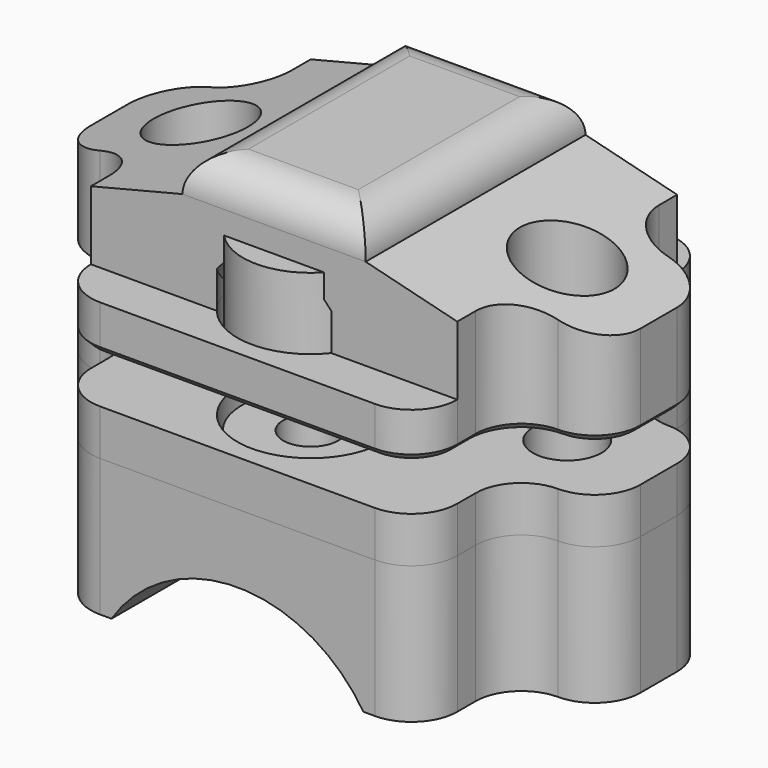
from build123d import *

# Parameters (mm, degrees)
F0_R      = 4.7625
F1_DEPTH  = 25.4
F3_DEPTH  = 63.5
F5_R      = 6.5405
F6_DEPTH  = 6.35
F9_DEPTH  = 12.7
F10_R     = 3.81
F10_R_2   = 4.7625
F11_DEPTH = 19.05
F12_R     = 3.81
F13_DEPTH = 4.445
F15_DEPTH = 63.5
F16_R     = 3.81
F17_DEPTH = 1.905
F20_R     = 4.7625
F21_DEPTH = 3.81
F22_R     = 6.5405
F23_DEPTH = 9.525
F24_R     = 6.5405
F25_DEPTH = 12.7
F27_DEPTH = 63.5
F29_DEPTH = 19.05
F30_R     = 7.62
F30_R_2   = 5.715
F31_DEPTH = 1.905
F32_R     = 5.07999
F33_R     = 3.175
F34_DEPTH = 21.59
F35_SIZE  = 0.889


# Not quite as in the source:
# - a fillet or chamfer is up to 0.001 mm smaller than in the source, because OpenCascade refuses the exact size
# - a feature of the source that left no trace in its solid (it failed there, or was rolled back) is left out


with BuildPart() as f1:
    # F0 (on Top) → F1 (new body)
    with BuildSketch(Plane.XY):
        with BuildLine():
            ThreePointArc((31.75, -9.525), (36.2401280605, -7.6651280605), (38.1, -3.175))
            Line((38.1, -3.175), (38.1, 3.175))
            ThreePointArc((38.1, 3.175), (36.2401280605, 7.6651280605), (31.75, 9.525))
            ThreePointArc((31.75, 9.525), (27.2598719395, 11.3848719395), (25.4, 15.875))
            Line((25.4, 15.875), (25.4, 19.05))
            ThreePointArc((25.4, 19.05), (23.5401280605, 23.5401280605), (19.05, 25.4))
            Line((19.05, 25.4), (-19.05, 25.4))
            ThreePointArc((-19.05, 25.4), (-23.5401280605, 23.5401280605), (-25.4, 19.05))
            Line((-25.4, 19.05), (-25.4, 15.875))
            ThreePointArc((-25.4, 15.875), (-27.2598719395, 11.3848719395), (-31.75, 9.525))
            ThreePointArc((-31.75, 9.525), (-36.2401280605, 7.6651280605), (-38.1, 3.175))
            Line((-38.1, 3.175), (-38.1, -3.175))
            ThreePointArc((-38.1, -3.175), (-36.2401280605, -7.6651280605), (-31.75, -9.525))
            ThreePointArc((-31.75, -9.525), (-27.2598719395, -11.3848719395), (-25.4, -15.875))
            Line((-25.4, -15.875), (-25.4, -19.05))
            ThreePointArc((-25.4, -19.05), (-23.5401280605, -23.5401280605), (-19.05, -25.4))
            Line((-19.05, -25.4), (19.05, -25.4))
            ThreePointArc((19.05, -25.4), (23.5401280605, -23.5401280605), (25.4, -19.05))
            Line((25.4, -19.05), (25.4, -15.875))
            ThreePointArc((25.4, -15.875), (27.2598719395, -11.3848719395), (31.75, -9.525))
        make_face()
        with Locations((-25.4, 0)):
            Circle(F0_R, mode=Mode.SUBTRACT)
        with BuildLine():
            ThreePointArc((-8.4822018349, 7.1073394495), (0, 22.86), (8.4822018349, 7.1073394495))
            ThreePointArc((8.4822018349, 7.1073394495), (6.35, 0), (8.4822018349, -7.1073394495))
            ThreePointArc((8.4822018349, -7.1073394495), (0, -22.86), (-8.4822018349, -7.1073394495))
            ThreePointArc((-8.4822018349, -7.1073394495), (-6.35, 0), (-8.4822018349, 7.1073394495))
        make_face(mode=Mode.SUBTRACT)
        with Locations((25.4, 0)):
            Circle(F0_R, mode=Mode.SUBTRACT)
    extrude(amount=F1_DEPTH)

    # F2 (on Front) → F3 (cut, symmetric)
    with BuildSketch(Plane.XZ):
        with BuildLine():
            Line((-19.05, -19.05), (19.05, -19.05))
            Line((19.05, -19.05), (19.05, 12.7))
            ThreePointArc((19.05, 12.7), (17.1901280605, 17.1901280605), (12.7, 19.05))
            Line((12.7, 19.05), (-12.7, 19.05))
            ThreePointArc((-12.7, 19.05), (-17.1901280605, 17.1901280605), (-19.05, 12.7))
            Line((-19.05, 12.7), (-19.05, -19.05))
        make_face()
    extrude(amount=F3_DEPTH, both=True, mode=Mode.SUBTRACT)


with BuildPart() as f6:
    # F5 (on offset) → F6 (new body)
    with BuildSketch(Plane.XY.offset(31.75)):
        with BuildLine():
            Line((-25.4, 19.05), (-25.4, 15.875))
            ThreePointArc((-25.4, 15.875), (-27.2598719395, 11.3848719395), (-31.75, 9.525))
            ThreePointArc((-31.75, 9.525), (-36.2401280605, 7.6651280605), (-38.1, 3.175))
            Line((-38.1, 3.175), (-38.1, -3.175))
            ThreePointArc((-38.1, -3.175), (-36.2401280605, -7.6651280605), (-31.75, -9.525))
            ThreePointArc((-31.75, -9.525), (-27.2598719395, -11.3848719395), (-25.4, -15.875))
            Line((-25.4, -15.875), (-25.4, -19.05))
            ThreePointArc((-25.4, -19.05), (-23.5401280605, -23.5401280605), (-19.05, -25.4))
            Line((-19.05, -25.4), (19.05, -25.4))
            ThreePointArc((19.05, -25.4), (23.5401280605, -23.5401280605), (25.4, -19.05))
            Line((25.4, -19.05), (25.4, -15.875))
            ThreePointArc((25.4, -15.875), (27.2598719395, -11.3848719395), (31.75, -9.525))
            ThreePointArc((31.75, -9.525), (36.2401280605, -7.6651280605), (38.1, -3.175))
            Line((38.1, -3.175), (38.1, 3.175))
            ThreePointArc((38.1, 3.175), (36.2401280605, 7.6651280605), (31.75, 9.525))
            ThreePointArc((31.75, 9.525), (27.2598719395, 11.3848719395), (25.4, 15.875))
            Line((25.4, 15.875), (25.4, 19.05))
            ThreePointArc((25.4, 19.05), (23.5401280605, 23.5401280605), (19.05, 25.4))
            Line((19.05, 25.4), (-19.05, 25.4))
            ThreePointArc((-19.05, 25.4), (-23.5401280605, 23.5401280605), (-25.4, 19.05))
        make_face()
        with Locations((-25.4, 0)):
            Circle(F5_R, mode=Mode.SUBTRACT)
        with BuildLine():
            ThreePointArc((-8.4822018349, 7.1073394495), (0, 22.86), (8.4822018349, 7.1073394495))
            ThreePointArc((8.4822018349, 7.1073394495), (6.35, 0), (8.4822018349, -7.1073394495))
            ThreePointArc((8.4822018349, -7.1073394495), (0, -22.86), (-8.4822018349, -7.1073394495))
            ThreePointArc((-8.4822018349, -7.1073394495), (-6.35, 0), (-8.4822018349, 7.1073394495))
        make_face(mode=Mode.SUBTRACT)
        with Locations((25.4, 0)):
            Circle(F5_R, mode=Mode.SUBTRACT)
    extrude(amount=F6_DEPTH)

    # F24 (on face) → F25 (join, through all)
    with BuildSketch(Plane.XY.offset(38.1)):
        with BuildLine():
            ThreePointArc((-25.4, 15.875), (-27.2598719395, 11.3848719395), (-31.75, 9.525))
            ThreePointArc((-31.75, 9.525), (-36.2401280605, 7.6651280605), (-38.1, 3.175))
            Line((-38.1, 3.175), (-38.1, -3.175))
            ThreePointArc((-38.1, -3.175), (-36.2401280605, -7.6651280605), (-31.75, -9.525))
            ThreePointArc((-31.75, -9.525), (-27.2598719395, -11.3848719395), (-25.4, -15.875))
            Line((-25.4, -15.875), (-25.4, -19.05))
            Line((-25.4, -19.05), (-7.931147458, -19.05))
            ThreePointArc((-7.931147458, -19.05), (-10.1492016439, -13.1683011766), (-8.4822018349, -7.1073394495))
            ThreePointArc((-8.4822018349, -7.1073394495), (-6.35, 0), (-8.4822018349, 7.1073394495))
            ThreePointArc((-8.4822018349, 7.1073394495), (-10.1492016439, 13.1683011766), (-7.931147458, 19.05))
            Line((-7.931147458, 19.05), (-25.4, 19.05))
            Line((-25.4, 19.05), (-25.4, 15.875))
        make_face()
        with Locations((-25.4, 0)):
            Circle(F24_R, mode=Mode.SUBTRACT)
        with BuildLine():
            Line((25.4, -19.05), (25.4, -15.875))
            ThreePointArc((25.4, -15.875), (27.2598719395, -11.3848719395), (31.75, -9.525))
            ThreePointArc((31.75, -9.525), (36.2401280605, -7.6651280605), (38.1, -3.175))
            Line((38.1, -3.175), (38.1, 3.175))
            ThreePointArc((38.1, 3.175), (36.2401280605, 7.6651280605), (31.75, 9.525))
            ThreePointArc((31.75, 9.525), (27.2598719395, 11.3848719395), (25.4, 15.875))
            Line((25.4, 15.875), (25.4, 19.05))
            Line((25.4, 19.05), (7.931147458, 19.05))
            ThreePointArc((7.931147458, 19.05), (10.1492016439, 13.1683011766), (8.4822018349, 7.1073394495))
            ThreePointArc((8.4822018349, 7.1073394495), (6.35, 0), (8.4822018349, -7.1073394495))
            ThreePointArc((8.4822018349, -7.1073394495), (10.1492016439, -13.1683011766), (7.931147458, -19.05))
            Line((7.931147458, -19.05), (25.4, -19.05))
        make_face()
        with Locations((25.4, 0)):
            Circle(F24_R, mode=Mode.SUBTRACT)
    extrude(amount=F25_DEPTH)

    # F26 (on Front) → F27 (cut, symmetric)
    with BuildSketch(Plane.XZ):
        Polygon((-38.1, 44.45), (-12.7, 50.8), (-38.1, 50.8), align=None)
        Polygon((38.1, 50.8), (12.7, 50.8), (38.1, 44.45), align=None)
    extrude(amount=F27_DEPTH, both=True, mode=Mode.SUBTRACT)



with BuildPart() as f9:
    # F8 (on offset) → F9 (new body)
    with BuildSketch(Plane.XY.offset(34.925)):
        with BuildLine():
            ThreePointArc((-7.8460366972, 7.5267889908), (-5.588, 0), (-7.8460366972, -7.5267889908))
            ThreePointArc((-7.8460366972, -7.5267889908), (0, -22.098), (7.8460366972, -7.5267889908))
            ThreePointArc((7.8460366972, -7.5267889908), (5.588, 0), (7.8460366972, 7.5267889908))
            ThreePointArc((7.8460366972, 7.5267889908), (0, 22.098), (-7.8460366972, 7.5267889908))
        make_face()
    extrude(amount=F9_DEPTH)


with BuildPart() as f11:
    # F10 (on Top) → F11 (new body)
    with BuildSketch(Plane.XY):
        with BuildLine():
            Line((19.05, 25.4), (-19.05, 25.4))
            ThreePointArc((-19.05, 25.4), (-23.5401280605, 23.5401280605), (-25.4, 19.05))
            Line((-25.4, 19.05), (-25.4, 15.875))
            ThreePointArc((-25.4, 15.875), (-27.2598719395, 11.3848719395), (-31.75, 9.525))
            ThreePointArc((-31.75, 9.525), (-36.2401280605, 7.6651280605), (-38.1, 3.175))
            Line((-38.1, 3.175), (-38.1, -3.175))
            ThreePointArc((-38.1, -3.175), (-36.2401280605, -7.6651280605), (-31.75, -9.525))
            ThreePointArc((-31.75, -9.525), (-27.2598719395, -11.3848719395), (-25.4, -15.875))
            Line((-25.4, -15.875), (-25.4, -19.05))
            ThreePointArc((-25.4, -19.05), (-23.5401280605, -23.5401280605), (-19.05, -25.4))
            Line((-19.05, -25.4), (19.05, -25.4))
            ThreePointArc((19.05, -25.4), (23.5401280605, -23.5401280605), (25.4, -19.05))
            Line((25.4, -19.05), (25.4, -15.875))
            ThreePointArc((25.4, -15.875), (27.2598719395, -11.3848719395), (31.75, -9.525))
            ThreePointArc((31.75, -9.525), (36.2401280605, -7.6651280605), (38.1, -3.175))
            Line((38.1, -3.175), (38.1, 3.175))
            ThreePointArc((38.1, 3.175), (36.2401280605, 7.6651280605), (31.75, 9.525))
            ThreePointArc((31.75, 9.525), (27.2598719395, 11.3848719395), (25.4, 15.875))
            Line((25.4, 15.875), (25.4, 19.05))
            ThreePointArc((25.4, 19.05), (23.5401280605, 23.5401280605), (19.05, 25.4))
        make_face()
        with Locations((0, -12.7)):
            Circle(F10_R, mode=Mode.SUBTRACT)
        with Locations((-25.4, 0)):
            Circle(F10_R_2, mode=Mode.SUBTRACT)
        with Locations((25.4, 0)):
            Circle(F10_R_2, mode=Mode.SUBTRACT)
        with Locations((0, 12.7)):
            Circle(F10_R, mode=Mode.SUBTRACT)
    extrude(amount=F11_DEPTH)

    # F12 (on face) → F13 (join)
    with BuildSketch(Plane.XY.offset(19.05)):
        with BuildLine():
            ThreePointArc((-7.9520642202, 7.4568807339), (-5.715, 0), (-7.9520642202, -7.4568807339))
            ThreePointArc((-7.9520642202, -7.4568807339), (0, -22.225), (7.9520642202, -7.4568807339))
            ThreePointArc((7.9520642202, -7.4568807339), (5.715, 0), (7.9520642202, 7.4568807339))
            ThreePointArc((7.9520642202, 7.4568807339), (0, 22.225), (-7.9520642202, 7.4568807339))
        make_face()
        with Locations((0, -12.7)):
            Circle(F12_R, mode=Mode.SUBTRACT)
        with Locations((0, 12.7)):
            Circle(F12_R, mode=Mode.SUBTRACT)
    extrude(amount=F13_DEPTH)

    # F14 (on Front) → F15 (cut, symmetric)
    with BuildSketch(Plane.XZ):
        with BuildLine():
            Line((-17.4625, 0), (17.4625, 0))
            ThreePointArc((17.4625, 0), (0, 9.525), (-17.4625, 0))
        make_face()
    extrude(amount=F15_DEPTH, both=True, mode=Mode.SUBTRACT)

    # F22 (on face) → F23 (cut)
    with BuildSketch(Plane.XY.offset(19.05)):
        with Locations((25.4, 0)):
            Circle(F22_R)
        with Locations((-25.4, 0)):
            Circle(F22_R)
    extrude(amount=-F23_DEPTH, mode=Mode.SUBTRACT)


with BuildPart() as f17:
    # F16 (on face) → F17 (new body)
    with BuildSketch(Plane(origin=(0, 0, 31.75), x_dir=(1, 0, 0), z_dir=(0, 0, -1))):
        with BuildLine():
            ThreePointArc((-7.9520642202, -7.4568807339), (0, -22.225), (7.9520642202, -7.4568807339))
            ThreePointArc((7.9520642202, -7.4568807339), (5.715, 0), (7.9520642202, 7.4568807339))
            ThreePointArc((7.9520642202, 7.4568807339), (0, 22.225), (-7.9520642202, 7.4568807339))
            ThreePointArc((-7.9520642202, 7.4568807339), (-5.715, 0), (-7.9520642202, -7.4568807339))
        make_face()
        with Locations((0, -12.7)):
            Circle(F16_R, mode=Mode.SUBTRACT)
        with Locations((0, 12.7)):
            Circle(F16_R, mode=Mode.SUBTRACT)
    extrude(amount=-F17_DEPTH)

    # F30 (on face) → F31 (join)
    with BuildSketch(Plane.XY.offset(33.655)):
        with Locations((0, -12.7)):
            Circle(F30_R)
        with Locations((0, -12.7)):
            Circle(F30_R_2, mode=Mode.SUBTRACT)
        with Locations((0, 12.7)):
            Circle(F30_R)
        with Locations((0, 12.7)):
            Circle(F30_R_2, mode=Mode.SUBTRACT)
    extrude(amount=F31_DEPTH)


with BuildPart() as f21:
    # F20 (on face) → F21 (new body)
    with BuildSketch(Plane.XY.offset(46.99)):
        with Locations((0, -12.7)):
            Circle(F20_R)
    extrude(amount=F21_DEPTH)


with BuildPart() as f21b:
    # F20 (on face) → F21, piece 2 (new body)
    with BuildSketch(Plane.XY.offset(46.99)):
        with Locations((0, 12.7)):
            Circle(F20_R)
    extrude(amount=F21_DEPTH)


with BuildPart() as f6_1:
    add(f6.part)

    add(f21.part)  # F29 merges F21

    add(f21b.part)  # F29 merges F21b
    # F28 (on Front) → F29 (join, symmetric)
    with BuildSketch(Plane.XZ):
        with BuildLine():
            ThreePointArc((-10.1854, 38.1), (0, 46.99), (10.1854, 38.1))
            Line((10.1854, 38.1), (12.7, 38.1))
            Line((12.7, 38.1), (12.7, 50.8))
            Line((12.7, 50.8), (12.7, 55.88))
            Line((12.7, 55.88), (-12.7, 55.88))
            Line((-12.7, 55.88), (-12.7, 50.8))
            Line((-12.7, 50.8), (-12.7, 38.1))
            Line((-12.7, 38.1), (-10.1854, 38.1))
        make_face()
    extrude(amount=F29_DEPTH, both=True)

    # F32 (radius 5.08 in the source; OpenCascade refuses exactly that, so slightly less here)
    f32_edges = [f6_1.edges().sort_by_distance(p)[0] for p in [
        (12.7, 0, 55.88),
        (0, 19.05, 55.88),
        (-12.7, 0, 55.88),
        (0, -19.05, 55.88),
    ]]
    fillet(f32_edges, radius=F32_R)

    # F33 (on face) → F34 (cut)
    with BuildSketch(Plane(origin=(0, 0, 31.75), x_dir=(1, 0, 0), z_dir=(0, 0, -1))):
        with Locations((0, 12.7)):
            Circle(F33_R)
        with Locations((0, -12.7)):
            Circle(F33_R)
    extrude(amount=-F34_DEPTH, mode=Mode.SUBTRACT)

    # F35
    f35_edges = [f6_1.edges().sort_by_distance(p)[0] for p in [
        (36.240128, -7.665128, 31.75),
        (38.1, 0, 31.75),
        (36.240128, 7.665128, 31.75),
        (27.259872, 11.384872, 31.75),
        (25.4, 17.4625, 31.75),
        (23.540128, 23.540128, 31.75),
        (0, 25.4, 31.75),
        (-23.540128, 23.540128, 31.75),
        (-25.4, 17.4625, 31.75),
        (-27.259872, 11.384872, 31.75),
        (-36.240128, 7.665128, 31.75),
        (-38.1, 0, 31.75),
        (-36.240128, -7.665128, 31.75),
        (-27.259872, -11.384872, 31.75),
        (-25.4, -17.4625, 31.75),
        (-23.540128, -23.540128, 31.75),
        (0, -25.4, 31.75),
        (23.540128, -23.540128, 31.75),
        (25.4, -17.4625, 31.75),
        (27.259872, -11.384872, 31.75),
        (-31.9405, 0, 31.75),
        (-6.35, 0, 31.75),
        (0, 22.86, 31.75),
        (6.35, 0, 31.75),
        (0, -22.86, 31.75),
        (18.8595, 0, 31.75),
    ]]
    chamfer(f35_edges, length=F35_SIZE)


solid = Compound([f1.part, f9.part, f11.part, f17.part, f6_1.part])
